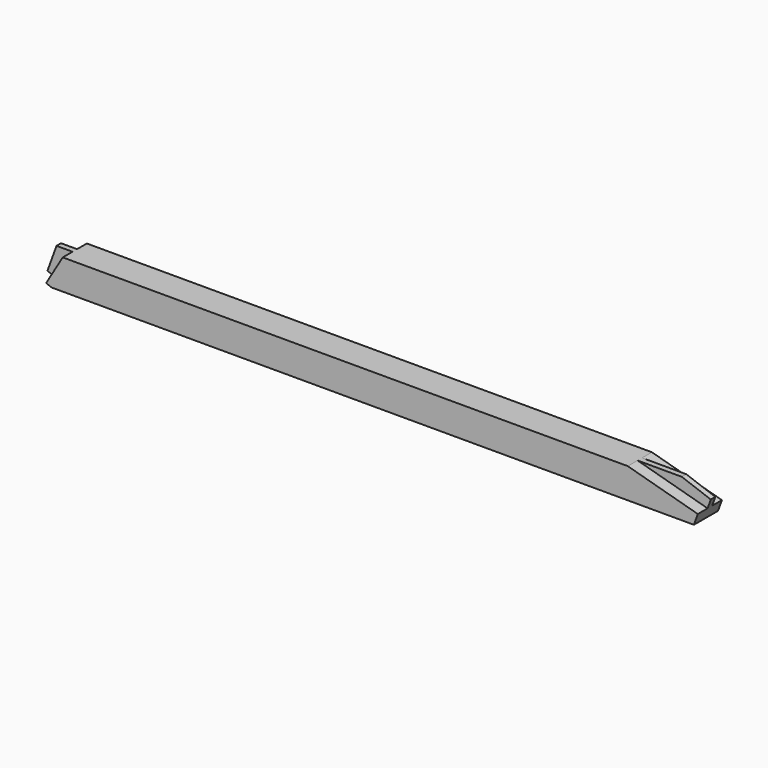
from build123d import *

# Parameters (mm, degrees)
F1_DEPTH = 101.6
F2_DEPTH = 19.05


with BuildPart() as f1:
    # F0 (on Front) → F1 (new body, symmetric)
    with BuildSketch(Plane.XZ):
        Polygon((1843.7016355094, 101.6), (-1966.2983644906, 101.6), (-1966.2983644906, -101.6), (2289.5986355094, -101.6), (2302.8887772145, -64.9607405868), (1948.7385730094, 63.5), (1909.5294683228, 77.7223004984), align=None)
        Polygon((-1966.2983644906, -101.6), (-1966.2983644906, 101.6), (-2040.0091644906, -101.6), align=None)
        Polygon((-2040.0091644906, -101.6), (-1966.2983644906, 101.6), (-2078.5961114712, -87.6025849828), align=None)
        Polygon((2315.8804976416, -29.1441913344), (1981.2986825646, 63.5), (1948.7385730094, 63.5), (2302.8887772145, -64.9607405868), align=None)
        Polygon((1981.2986825646, 63.5), (1843.7016355094, 101.6), (1909.5294683228, 77.7223004984), (1948.7385730094, 63.5), align=None)
    extrude(amount=F1_DEPTH, both=True)

    # F0 (on Front) → F2 (join, symmetric)
    with BuildSketch(Plane.XZ):
        Polygon((-1966.2983644906, 101.6), (-2074.3764867409, 101.6), (-2135.519336069, -66.9536852599), (-2078.5961114712, -87.6025849828), align=None)
        Polygon((1981.2986825646, 63.5), (1843.7016355094, 101.6), (1909.5294683228, 77.7223004984), (1948.7385730094, 63.5), align=None)
        Polygon((1918.1906152742, 101.6), (1843.7016355094, 101.6), (1981.2986825646, 63.5), (2246.6944920684, 63.5), (2141.6575545684, 101.6), align=None)
        Polygon((2315.8804976416, -29.1441913344), (1981.2986825646, 63.5), (1948.7385730094, 63.5), (2302.8887772145, -64.9607405868), align=None)
        Polygon((2246.6944920684, 63.5), (1981.2986825646, 63.5), (2315.8804976416, -29.1441913344), (2337.53336502, 30.5500574195), align=None)
    extrude(amount=F2_DEPTH, both=True)


solid = f1.part
